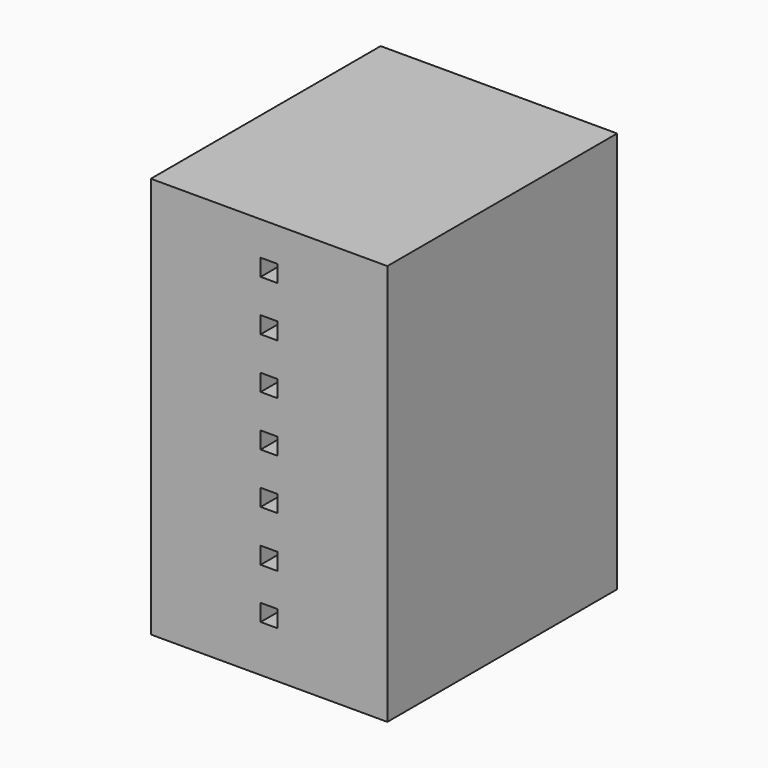
from build123d import *

# Parameters (mm, degrees)
F1_DEPTH      = 431.8
F2_W          = 152.4
F2_H          = 50.8
F3_DEPTH      = 381
F4_DEPTH      = 381
F6_DEPTH      = 256.54
F7_DEPTH      = 228.6
F8_DEPTH      = 482.6
F9_DEPTH      = 284.48
F10_DEPTH     = 259.842
F11_DEPTH     = 279.4
F12_DEPTH     = 254
F13_DEPTH     = 254
F15_DEPTH     = 25.4
F16_DEPTH     = 25.4
F17_DEPTH     = 25.4
F14_W         = 4.9380194978
F14_H         = 46.2689572596
F18_DEPTH     = 25.4
F14_TEXT_SIZE = 55.4215783874
F19_DEPTH     = 25.4


# Not quite as in the source:
# - Text() gives the source's letters only with a copy of the font that has no kerning and outlines rounded to 1/6400 em; it was checked with that copy


with BuildPart() as f1:
    # F0 (on Front) → F1 (new body)
    with BuildSketch(Plane.XZ):
        Polygon((0, 0), (0, -301.625), (177.8, -301.625), (177.8, 301.625), (0, 301.625), align=None)
        Polygon((-177.8, -301.625), (0, -301.625), (0, 0), (0, 301.625), (-177.8, 301.625), align=None)
    extrude(amount=F1_DEPTH)

    # F2 (on face) → F3 (cut)
    with BuildSketch(Plane(origin=(0, 0, 0), x_dir=(-1, 0, 0), z_dir=(0, 1, 0))):
        with Locations((-76.2, 98.425)):
            Rectangle(F2_W, F2_H)
        with Locations((-76.2, 22.225)):
            Rectangle(F2_W, F2_H)
        with Locations((-76.2, -53.975)):
            Rectangle(F2_W, F2_H)
        with Locations((-76.2, -130.175)):
            Rectangle(F2_W, F2_H)
        with Locations((-76.2, -206.375)):
            Rectangle(F2_W, F2_H)
        with Locations((-76.2, 174.625)):
            Rectangle(F2_W, F2_H)
        with Locations((-76.2, 250.825)):
            Rectangle(F2_W, F2_H)
    extrude(amount=-F3_DEPTH, mode=Mode.SUBTRACT)

    # F2 (on face) → F4 (cut)
    with BuildSketch(Plane(origin=(0, 0, 0), x_dir=(-1, 0, 0), z_dir=(0, 1, 0))):
        with Locations((76.2, 250.825)):
            Rectangle(F2_W, F2_H)
        with Locations((76.2, 174.625)):
            Rectangle(F2_W, F2_H)
        with Locations((76.2, 98.425)):
            Rectangle(F2_W, F2_H)
        with Locations((76.2, 22.225)):
            Rectangle(F2_W, F2_H)
        with Locations((76.2, -53.975)):
            Rectangle(F2_W, F2_H)
        with Locations((76.2, -130.175)):
            Rectangle(F2_W, F2_H)
        with Locations((76.2, -206.375)):
            Rectangle(F2_W, F2_H)
    extrude(amount=-F4_DEPTH, mode=Mode.SUBTRACT)

    # F5 (on face) → F6 (cut)
    with BuildSketch(Plane(origin=(0, -381, 0), x_dir=(-1, 0, 0), z_dir=(0, 1, 0))):
        Polygon((-12.7, 225.425), (0, 225.425), (12.7, 225.425), (12.7, 250.825), (-12.7, 250.825), align=None)
    extrude(amount=-F6_DEPTH, mode=Mode.SUBTRACT)

    # F5 (on face) → F7 (cut)
    with BuildSketch(Plane(origin=(0, -381, 0), x_dir=(-1, 0, 0), z_dir=(0, 1, 0))):
        Polygon((-12.7, 73.0780788422), (0, 73.0780788422), (12.7, 73.0780788422), (12.7, 98.4780788422), (-12.7, 98.4780788422), align=None)
    extrude(amount=-F7_DEPTH, mode=Mode.SUBTRACT)

    # F5 (on face) → F8 (cut)
    with BuildSketch(Plane(origin=(0, -381, 0), x_dir=(-1, 0, 0), z_dir=(0, 1, 0))):
        Polygon((-12.7, 149.3929922581), (0, 149.3929922581), (12.7, 149.3929922581), (12.7, 174.7929922581), (-12.7, 174.7929922581), align=None)
    extrude(amount=F8_DEPTH, mode=Mode.SUBTRACT)

    # F5 (on face) → F9 (cut)
    with BuildSketch(Plane(origin=(0, -381, 0), x_dir=(-1, 0, 0), z_dir=(0, 1, 0))):
        Polygon((-12.7, 149.3929922581), (0, 149.3929922581), (12.7, 149.3929922581), (12.7, 174.7929922581), (-12.7, 174.7929922581), align=None)
    extrude(amount=-F9_DEPTH, mode=Mode.SUBTRACT)

    # F5 (on face) → F10 (cut)
    with BuildSketch(Plane(origin=(0, -381, 0), x_dir=(-1, 0, 0), z_dir=(0, 1, 0))):
        Polygon((-12.7, -3.174306592), (0, -3.174306592), (12.7, -3.174306592), (12.7, 22.225693408), (-12.7, 22.225693408), align=None)
    extrude(amount=-F10_DEPTH, mode=Mode.SUBTRACT)

    # F5 (on face) → F11 (cut)
    with BuildSketch(Plane(origin=(0, -381, 0), x_dir=(-1, 0, 0), z_dir=(0, 1, 0))):
        Polygon((-12.7, -79.1038572788), (0, -79.1038572788), (12.7, -79.1038572788), (12.7, -53.7038572788), (-12.7, -53.7038572788), align=None)
    extrude(amount=-F11_DEPTH, mode=Mode.SUBTRACT)

    # F5 (on face) → F12 (cut)
    with BuildSketch(Plane(origin=(0, -381, 0), x_dir=(-1, 0, 0), z_dir=(0, 1, 0))):
        Polygon((-12.7, -155.6432694197), (0, -155.6432694197), (12.7, -155.6432694197), (12.7, -130.2432694197), (-12.7, -130.2432694197), align=None)
    extrude(amount=-F12_DEPTH, mode=Mode.SUBTRACT)

    # F5 (on face) → F13 (cut)
    with BuildSketch(Plane(origin=(0, -381, 0), x_dir=(-1, 0, 0), z_dir=(0, 1, 0))):
        Polygon((-12.7, -231.3715964556), (0, -231.3715964556), (12.7, -231.3715964556), (12.7, -205.9715964556), (-12.7, -205.9715964556), align=None)
    extrude(amount=-F13_DEPTH, mode=Mode.SUBTRACT)

    # F14 (on face) → F15 (cut)
    with BuildSketch(Plane(origin=(0, 0, 0), x_dir=(-1, 0, 0), z_dir=(0, 1, 0))):
        Polygon((-140.4538663919, -265.5288285071), (-135.0401224724, -279.3533802032), (-129.8071538331, -279.3533802032), (-146.9046895509, -235.7009072633), (-151.1576658813, -235.7009072633), (-168.340831995, -279.3533802032), (-163.222037217, -279.3533802032), (-157.8748947165, -265.5288285071), align=None)
        with BuildLine():
            Line((-147.0854648311, -247.5083874112), (-142.0237569837, -260.9809030352))
            Line((-142.0237569837, -260.9809030352), (-156.0861708907, -260.9809030352))
            Line((-156.0861708907, -260.9809030352), (-150.9768906011, -247.5083874112))
            add(Edge.make_bspline(
                [(-149.1025363794, -241.2383395325), (-149.7590360814, -244.092686063), (-150.9768906011, -247.5083874112)],
                knots=[0, 0, 0, 1, 1, 1], degree=2))
            add(Edge.make_bspline(
                [(-147.0854648311, -247.5083874112), (-148.0654571399, -244.9489900221), (-149.1025363794, -241.2383395325)],
                knots=[0, 0, 0, 1, 1, 1], degree=2))
        make_face(mode=Mode.SUBTRACT)
    extrude(amount=-F15_DEPTH, mode=Mode.SUBTRACT)

    # F14 (on face) → F16 (cut)
    with BuildSketch(Plane(origin=(0, 0, 0), x_dir=(-1, 0, 0), z_dir=(0, 1, 0))):
        with BuildLine():
            Line((-124.5741851938, -246.7662573132), (-124.5741851938, -279.3533802032))
            Line((-124.5741851938, -279.3533802032), (-120.8733394742, -279.3533802032))
            Line((-120.8733394742, -279.3533802032), (-119.636165696, -279.3533802032))
            Line((-119.636165696, -279.3533802032), (-119.636165696, -262.2558444855))
            add(Edge.make_bspline(
                [(-117.2575435873, -253.1266928321), (-119.636165696, -255.8906517224), (-119.636165696, -262.2558444855)],
                knots=[0, 0, 0, 1, 1, 1], degree=2))
            add(Edge.make_bspline(
                [(-109.7696411889, -250.3627339417), (-114.8789214785, -250.3627339417), (-117.2575435873, -253.1266928321)],
                knots=[0, 0, 0, 1, 1, 1], degree=2))
            add(Edge.make_bspline(
                [(-104.084734349, -252.3274758035), (-105.8972443958, -250.3627339417), (-109.7696411889, -250.3627339417)],
                knots=[0, 0, 0, 1, 1, 1], degree=2))
            add(Edge.make_bspline(
                [(-102.2722243021, -258.2692738312), (-102.2722243021, -254.2922176654), (-104.084734349, -252.3274758035)],
                knots=[0, 0, 0, 1, 1, 1], degree=2))
            Line((-102.2722243021, -258.2692738312), (-102.2722243021, -279.3533802032))
            Line((-102.2722243021, -279.3533802032), (-98.6330062151, -279.3533802032))
            Line((-98.6330062151, -279.3533802032), (-97.3342048043, -279.3533802032))
            Line((-97.3342048043, -279.3533802032), (-97.3342048043, -258.0980130394))
            add(Edge.make_bspline(
                [(-100.3074824403, -249.0069193397), (-97.3342048043, -251.8469941375), (-97.3342048043, -258.0980130394)],
                knots=[0, 0, 0, 1, 1, 1], degree=2))
            add(Edge.make_bspline(
                [(-109.1702284175, -246.1668445418), (-103.2807600762, -246.1668445418), (-100.3074824403, -249.0069193397)],
                knots=[0, 0, 0, 1, 1, 1], degree=2))
            add(Edge.make_bspline(
                [(-115.2642582601, -247.4941156785), (-112.5288428351, -246.1668445418), (-109.1702284175, -246.1668445418)],
                knots=[0, 0, 0, 1, 1, 1], degree=2))
            add(Edge.make_bspline(
                [(-119.5219918348, -251.2285523893), (-117.9996736852, -248.8213868152), (-115.2642582601, -247.4941156785)],
                knots=[0, 0, 0, 1, 1, 1], degree=2))
            Line((-119.5219918348, -251.2285523893), (-119.7598540457, -251.2285523893))
            Line((-119.7598540457, -251.2285523893), (-120.5590710742, -246.7662573132))
            Line((-120.5590710742, -246.7662573132), (-124.5741851938, -246.7662573132))
        make_face()
    extrude(amount=-F16_DEPTH, mode=Mode.SUBTRACT)

    # F14 (on face) → F17 (cut)
    with BuildSketch(Plane(origin=(0, 0, 0), x_dir=(-1, 0, 0), z_dir=(0, 1, 0))):
        with BuildLine():
            Line((-60.5321635376, -249.8870095199), (-60.5321635376, -246.7662573132))
            Line((-60.5321635376, -246.7662573132), (-71.7973178447, -246.7662573132))
            add(Edge.make_bspline(
                [(-76.4118447357, -246.1668445418), (-73.8524473466, -246.1668445418), (-71.7973178447, -246.7662573132)],
                knots=[0, 0, 0, 1, 1, 1], degree=2))
            add(Edge.make_bspline(
                [(-85.5029384353, -249.0687635145), (-82.2917985885, -246.1668445418), (-76.4118447357, -246.1668445418)],
                knots=[0, 0, 0, 1, 1, 1], degree=2))
            add(Edge.make_bspline(
                [(-88.7140782822, -257.3178249877), (-88.7140782822, -251.9706824872), (-85.5029384353, -249.0687635145)],
                knots=[0, 0, 0, 1, 1, 1], degree=2))
            add(Edge.make_bspline(
                [(-87.1251587135, -263.0312752929), (-88.7140782822, -260.5337220787), (-88.7140782822, -257.3178249877)],
                knots=[0, 0, 0, 1, 1, 1], degree=2))
            add(Edge.make_bspline(
                [(-83.0053852211, -266.5659077466), (-85.5362391449, -265.5288285071), (-87.1251587135, -263.0312752929)],
                knots=[0, 0, 0, 1, 1, 1], degree=2))
            add(Edge.make_bspline(
                [(-86.0119635666, -269.1538486009), (-85.0605147231, -267.8123057315), (-83.0053852211, -266.5659077466)],
                knots=[0, 0, 0, 1, 1, 1], degree=2))
            add(Edge.make_bspline(
                [(-86.9634124101, -272.2746008076), (-86.9634124101, -270.4953914702), (-86.0119635666, -269.1538486009)],
                knots=[0, 0, 0, 1, 1, 1], degree=2))
            add(Edge.make_bspline(
                [(-86.1166229394, -275.0433169422), (-86.9634124101, -273.8540058878), (-86.9634124101, -272.2746008076)],
                knots=[0, 0, 0, 1, 1, 1], degree=2))
            add(Edge.make_bspline(
                [(-84.0234354837, -276.7939828142), (-85.2698334687, -276.2326279966), (-86.1166229394, -275.0433169422)],
                knots=[0, 0, 0, 1, 1, 1], degree=2))
            add(Edge.make_bspline(
                [(-89.3705779842, -279.7387169849), (-87.4676802972, -277.5646563775), (-84.0234354837, -276.7939828142)],
                knots=[0, 0, 0, 1, 1, 1], degree=2))
            add(Edge.make_bspline(
                [(-91.2734756712, -284.881297984), (-91.2734756712, -281.9127775923), (-89.3705779842, -279.7387169849)],
                knots=[0, 0, 0, 1, 1, 1], degree=2))
            add(Edge.make_bspline(
                [(-87.8102018808, -291.6080413076), (-91.2734756712, -289.2294191988), (-91.2734756712, -284.881297984)],
                knots=[0, 0, 0, 1, 1, 1], degree=2))
            add(Edge.make_bspline(
                [(-77.9531918621, -293.9866634163), (-84.3469280905, -293.9866634163), (-87.8102018808, -291.6080413076)],
                knots=[0, 0, 0, 1, 1, 1], degree=2))
            add(Edge.make_bspline(
                [(-65.2894077551, -291.1465886185), (-69.6280144815, -293.9866634163), (-77.9531918621, -293.9866634163)],
                knots=[0, 0, 0, 1, 1, 1], degree=2))
            add(Edge.make_bspline(
                [(-60.9508010287, -282.8927699011), (-60.9508010287, -288.3065138206), (-65.2894077551, -291.1465886185)],
                knots=[0, 0, 0, 1, 1, 1], degree=2))
            add(Edge.make_bspline(
                [(-63.7861185824, -276.4086460326), (-60.9508010287, -278.6397935706), (-60.9508010287, -282.8927699011)],
                knots=[0, 0, 0, 1, 1, 1], degree=2))
            add(Edge.make_bspline(
                [(-71.9210061943, -274.1774984946), (-66.621436136, -274.1774984946), (-63.7861185824, -276.4086460326)],
                knots=[0, 0, 0, 1, 1, 1], degree=2))
            Line((-71.9210061943, -274.1774984946), (-77.686786186, -274.1774984946))
            add(Edge.make_bspline(
                [(-81.4592808504, -273.5400277694), (-80.3603574362, -274.1774984946), (-77.686786186, -274.1774984946)],
                knots=[0, 0, 0, 1, 1, 1], degree=2))
            add(Edge.make_bspline(
                [(-82.5582042647, -271.5610141749), (-82.5582042647, -272.9025570443), (-81.4592808504, -273.5400277694)],
                knots=[0, 0, 0, 1, 1, 1], degree=2))
            add(Edge.make_bspline(
                [(-79.4089085927, -267.3746392635), (-82.5582042647, -269.0396747397), (-82.5582042647, -271.5610141749)],
                knots=[0, 0, 0, 1, 1, 1], degree=2))
            add(Edge.make_bspline(
                [(-76.6782504118, -267.6125014744), (-78.1339671424, -267.6125014744), (-79.4089085927, -267.3746392635)],
                knots=[0, 0, 0, 1, 1, 1], degree=2))
            add(Edge.make_bspline(
                [(-67.6965733292, -264.7581549439), (-70.9695573508, -267.6125014744), (-76.6782504118, -267.6125014744)],
                knots=[0, 0, 0, 1, 1, 1], degree=2))
            add(Edge.make_bspline(
                [(-64.4235893075, -257.1085062421), (-64.4235893075, -261.9038084134), (-67.6965733292, -264.7581549439)],
                knots=[0, 0, 0, 1, 1, 1], degree=2))
            add(Edge.make_bspline(
                [(-65.0800890095, -253.321739845), (-64.4235893075, -255.005804298), (-64.4235893075, -257.1085062421)],
                knots=[0, 0, 0, 1, 1, 1], degree=2))
            add(Edge.make_bspline(
                [(-66.5643492054, -250.6005961526), (-65.7365887115, -251.637675392), (-65.0800890095, -253.321739845)],
                knots=[0, 0, 0, 1, 1, 1], degree=2))
            Line((-66.5643492054, -250.6005961526), (-60.5321635376, -249.8870095199))
        make_face()
        with BuildLine():
            add(Edge.make_bspline(
                [(-86.5162314537, -284.8242110534), (-86.5162314537, -287.4692388383), (-84.2850839157, -288.839325173)],
                knots=[0, 0, 0, 1, 1, 1], degree=2))
            add(Edge.make_bspline(
                [(-84.641877232, -280.2144414066), (-86.5162314537, -281.8176327079), (-86.5162314537, -284.8242110534)],
                knots=[0, 0, 0, 1, 1, 1], degree=2))
            add(Edge.make_bspline(
                [(-79.4089085927, -278.6112501053), (-82.7675230103, -278.6112501053), (-84.641877232, -280.2144414066)],
                knots=[0, 0, 0, 1, 1, 1], degree=2))
            Line((-79.4089085927, -278.6112501053), (-73.4908967861, -278.6112501053))
            add(Edge.make_bspline(
                [(-67.3397800128, -279.6388148563), (-68.9715147795, -278.6112501053), (-73.4908967861, -278.6112501053)],
                knots=[0, 0, 0, 1, 1, 1], degree=2))
            add(Edge.make_bspline(
                [(-65.7080452462, -283.3114073922), (-65.7080452462, -280.6663796073), (-67.3397800128, -279.6388148563)],
                knots=[0, 0, 0, 1, 1, 1], degree=2))
            add(Edge.make_bspline(
                [(-68.6955946148, -288.3493290186), (-65.7080452462, -286.4892465295), (-65.7080452462, -283.3114073922)],
                knots=[0, 0, 0, 1, 1, 1], degree=2))
            add(Edge.make_bspline(
                [(-77.8961049315, -290.2094115076), (-71.6831439834, -290.2094115076), (-68.6955946148, -288.3493290186)],
                knots=[0, 0, 0, 1, 1, 1], degree=2))
            add(Edge.make_bspline(
                [(-84.2850839157, -288.839325173), (-82.0539363776, -290.2094115076), (-77.8961049315, -290.2094115076)],
                knots=[0, 0, 0, 1, 1, 1], degree=2))
        make_face(mode=Mode.SUBTRACT)
        with BuildLine():
            add(Edge.make_bspline(
                [(-83.8426602034, -257.2036511265), (-83.8426602034, -260.6193524747), (-81.9112190511, -262.3747755909)],
                knots=[0, 0, 0, 1, 1, 1], degree=2))
            add(Edge.make_bspline(
                [(-81.9683059817, -251.6424326362), (-83.8426602034, -253.5120296137), (-83.8426602034, -257.2036511265)],
                knots=[0, 0, 0, 1, 1, 1], degree=2))
            add(Edge.make_bspline(
                [(-76.6116489928, -249.7728356587), (-80.09395176, -249.7728356587), (-81.9683059817, -251.6424326362)],
                knots=[0, 0, 0, 1, 1, 1], degree=2))
            add(Edge.make_bspline(
                [(-69.3045218747, -257.1085062421), (-69.3045218747, -249.7728356587), (-76.6116489928, -249.7728356587)],
                knots=[0, 0, 0, 1, 1, 1], degree=2))
            add(Edge.make_bspline(
                [(-76.5260185969, -264.1301987072), (-69.3045218747, -264.1301987072), (-69.3045218747, -257.1085062421)],
                knots=[0, 0, 0, 1, 1, 1], degree=2))
            add(Edge.make_bspline(
                [(-81.9112190511, -262.3747755909), (-79.9797778988, -264.1301987072), (-76.5260185969, -264.1301987072)],
                knots=[0, 0, 0, 1, 1, 1], degree=2))
        make_face(mode=Mode.SUBTRACT)
    extrude(amount=-F17_DEPTH, mode=Mode.SUBTRACT)

    # F14 (on face) → F18 (cut)
    with BuildSketch(Plane(origin=(0, 0, 0), x_dir=(-1, 0, 0), z_dir=(0, 1, 0))):
        with BuildLine():
            add(Edge.make_bspline(
                [(-40.0760134022, -279.9527929747), (-47.2975101244, -279.9527929747), (-51.4791277916, -275.5475848292)],
                knots=[0, 0, 0, 1, 1, 1], degree=2))
            add(Edge.make_bspline(
                [(-34.4434362487, -279.458039576), (-36.7744859153, -279.9527929747), (-40.0760134022, -279.9527929747)],
                knots=[0, 0, 0, 1, 1, 1], degree=2))
            add(Edge.make_bspline(
                [(-29.4959022625, -277.8405765421), (-32.1123865821, -278.9632861774), (-34.4434362487, -279.458039576)],
                knots=[0, 0, 0, 1, 1, 1], degree=2))
            Line((-29.4959022625, -277.8405765421), (-29.4959022625, -273.4353683967))
            add(Edge.make_bspline(
                [(-39.895238122, -275.6332152251), (-34.6337260174, -275.6332152251), (-29.4959022625, -273.4353683967)],
                knots=[0, 0, 0, 1, 1, 1], degree=2))
            add(Edge.make_bspline(
                [(-47.6400317081, -272.6599375892), (-44.8903445504, -275.6332152251), (-39.895238122, -275.6332152251)],
                knots=[0, 0, 0, 1, 1, 1], degree=2))
            add(Edge.make_bspline(
                [(-50.5419506808, -263.9494234269), (-50.3897188658, -269.6866599532), (-47.6400317081, -272.6599375892)],
                knots=[0, 0, 0, 1, 1, 1], degree=2))
            Line((-50.5419506808, -263.9494234269), (-28.0972724625, -263.9494234269))
            Line((-28.0972724625, -263.9494234269), (-28.0972724625, -260.8286712202))
            add(Edge.make_bspline(
                [(-31.6652056257, -250.1962303941), (-28.0972724625, -254.2256162463), (-28.0972724625, -260.8286712202)],
                knots=[0, 0, 0, 1, 1, 1], degree=2))
            add(Edge.make_bspline(
                [(-41.3509548525, -246.1668445418), (-35.2331387888, -246.1668445418), (-31.6652056257, -250.1962303941)],
                knots=[0, 0, 0, 1, 1, 1], degree=2))
            add(Edge.make_bspline(
                [(-51.7788341773, -250.8051576539), (-47.8969228958, -246.1668445418), (-41.3509548525, -246.1668445418)],
                knots=[0, 0, 0, 1, 1, 1], degree=2))
            add(Edge.make_bspline(
                [(-55.6607454588, -263.3309816786), (-55.6607454588, -255.443470766), (-51.7788341773, -250.8051576539)],
                knots=[0, 0, 0, 1, 1, 1], degree=2))
            add(Edge.make_bspline(
                [(-51.4791277916, -275.5475848292), (-55.6607454588, -271.1423766838), (-55.6607454588, -263.3309816786)],
                knots=[0, 0, 0, 1, 1, 1], degree=2))
        make_face()
        with BuildLine():
            add(Edge.make_bspline(
                [(-41.4175562716, -250.3056470111), (-45.3375255068, -250.3056470111), (-47.6733324176, -252.8602871559)],
                knots=[0, 0, 0, 1, 1, 1], degree=2))
            add(Edge.make_bspline(
                [(-35.4662437555, -252.7889284926), (-37.5451594785, -250.3056470111), (-41.4175562716, -250.3056470111)],
                knots=[0, 0, 0, 1, 1, 1], degree=2))
            add(Edge.make_bspline(
                [(-33.3873280324, -259.9343093073), (-33.3873280324, -255.2722099742), (-35.4662437555, -252.7889284926)],
                knots=[0, 0, 0, 1, 1, 1], degree=2))
            Line((-33.3873280324, -259.9343093073), (-50.4277768196, -259.9343093073))
            add(Edge.make_bspline(
                [(-47.6733324176, -252.8602871559), (-50.0091393284, -255.4149273007), (-50.4277768196, -259.9343093073)],
                knots=[0, 0, 0, 1, 1, 1], degree=2))
        make_face(mode=Mode.SUBTRACT)
        with Locations((-17.2079404486, -256.2189015734)):
            Rectangle(F14_W, F14_H)
    extrude(amount=-F18_DEPTH, mode=Mode.SUBTRACT)

    # F14 (on face) → F19 (cut)
    with BuildSketch(Plane(origin=(0, 0, 0), x_dir=(-1, 0, 0), z_dir=(0, 1, 0))):
        with Locations((8.155670017, -278.3586084843)):
            Text('E.', F14_TEXT_SIZE, font='Open Sans', text_align=(TextAlign.LEFT, TextAlign.BOTTOM))
    extrude(amount=-F19_DEPTH, mode=Mode.SUBTRACT)


solid = f1.part
